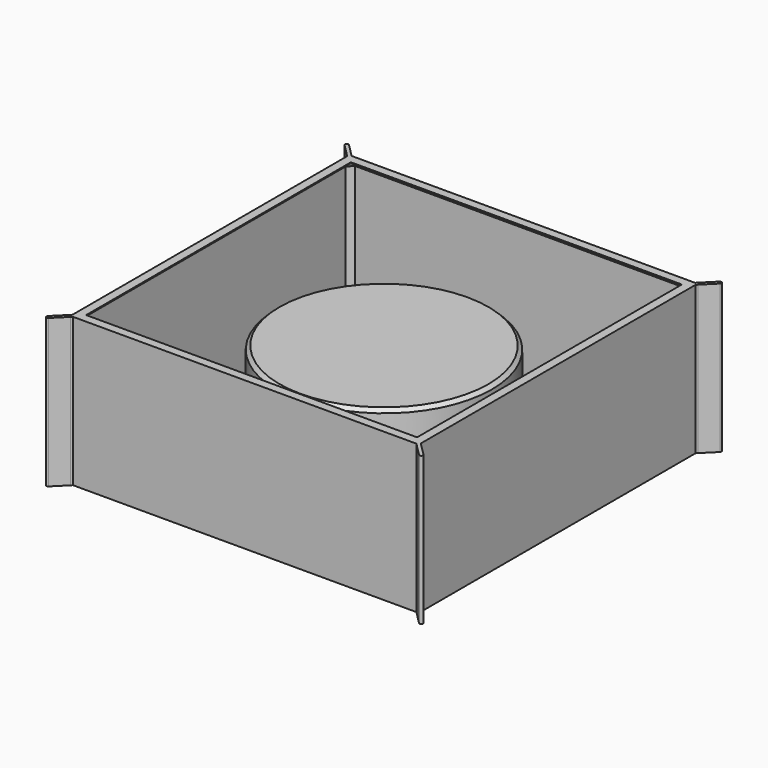
from build123d import *

# Parameters (mm, degrees)
F0_W             = 80
F0_H             = 80
F1_DEPTH         = 34
F2_T             = -0.8
F3_R             = 25
F4_DEPTH         = 24
F4_TAPER         = 0.5
F5_T1_DEPTH      = 78.4
F5_T3_DEPTH      = 78.4
F6_W             = 80
F6_H             = 80
F6_W_2           = 76
F6_H_2           = 76
F7_DEPTH         = 0.05
F8_SIZE          = 1.19999
F11_DEPTH        = 34.05
F11_COPIES_COUNT = 4


# Not quite as in the source:
# - a fillet or chamfer that OpenCascade refuses, or shapes differently, is made with other operations: its cross-section is extruded or revolved along the edge and cut away or added
# - a fillet or chamfer is up to 0.001 mm smaller than in the source, because OpenCascade refuses the exact size
# - a pattern or mirror of a feature is missing from the dataset's text; its kind, count and spacing are read off the source's solid


with BuildPart() as f1:
    # F0 (on Top) → F1 (new body)
    with BuildSketch(Plane.XY):
        Rectangle(F0_W, F0_H)
    extrude(amount=F1_DEPTH)

    # F2
    f2_openings = [f1.faces().sort_by_distance(p)[0] for p in [
        (0, 0, 34),
    ]]
    offset(amount=F2_T, openings=f2_openings)

    # F3 (on face) → F4 (join)
    with BuildSketch(Plane.XY.offset(0.8)):
        Circle(F3_R)
    extrude(amount=F4_DEPTH, taper=F4_TAPER)

    # F5: chamfer of 1.2 on 5 edges, made by hand

    # F5_s2 → F5_t1 (join)
    with BuildSketch(Plane.XZ.offset(-39.2)):
        Polygon((-39.2, 2), (-38, 0.8), (-39.2, 0.8), align=None)
        Polygon((39.2, 2), (38, 0.8), (39.2, 0.8), align=None)
    extrude(amount=F5_T1_DEPTH)

    # F5_s4 → F5_t3 (join)
    with BuildSketch(Plane.YZ.offset(-39.2)):
        Polygon((-39.2, 2), (-38, 0.8), (-39.2, 0.8), align=None)
        Polygon((39.2, 2), (38, 0.8), (39.2, 0.8), align=None)
    extrude(amount=F5_T3_DEPTH)

    # F5_s5 → F5_t6 (revolve)
    with BuildSketch(Plane.XZ):
        Polygon((26.1895734527, 0.8), (24.989619145, 1.9895281574), (25, 0.8), align=None)
    revolve(axis=Axis((0, 0, 0.8), (0, 0, -1)))

    # F6 (on face) → F7 (join)
    with BuildSketch(Plane.XY.offset(34)):
        Rectangle(F6_W, F6_H)
        Rectangle(F6_W_2, F6_H_2, mode=Mode.SUBTRACT)
    extrude(amount=F7_DEPTH)

    # F8 (size 1.2 in the source; OpenCascade refuses exactly that, so slightly less here)
    f8_edges = [f1.edges().sort_by_distance(p)[0] for p in [
        (0, -39.2, 34),
        (-39.2, 0, 34),
        (-39.2, -39.2, 18),
        (-39.2, 39.2, 18),
        (0, 39.2, 34),
        (39.2, 0, 34),
        (39.2, 39.2, 18),
        (39.2, -39.2, 18),
    ]]
    chamfer(f8_edges, length=F8_SIZE)

    # F9: chamfer of 0.8 on 1 edges, made by hand

    # F9_s1 → F9_t2 (revolve, cut)
    with BuildSketch(Plane.XZ):
        Polygon((24.7975364014, 24.0000304615), (23.990555173, 24.8), (24.790555173, 24.8), align=None)
    revolve(axis=Axis((0, 0, 24.8), (0, 0, -1)), mode=Mode.SUBTRACT)

    # F10 (on face) → F11 (join, through all)
    with BuildSketch(Plane(origin=(0, 0, 0), x_dir=(1, 0, 0), z_dir=(0, 0, -1))):
        with BuildLine():
            Line((-39.1612012219, 39.7268866468), (-39.7171572875, 40.2828427125))
            ThreePointArc((-39.7171572875, 40.2828427125), (-39.7171572875, 39.7171572875), (-40.2828427125, 39.7171572875))
            Line((-40.2828427125, 39.7171572875), (-39.7268866468, 39.1612012219))
            Line((-39.7268866468, 39.1612012219), (-39.1612012219, 39.7268866468))
        make_face()
        with BuildLine():
            ThreePointArc((-40.2828427125, 39.7171572875), (-39.7171572875, 39.7171572875), (-39.7171572875, 40.2828427125))
            Line((-39.7171572875, 40.2828427125), (-42.5455844123, 43.1112698372))
            ThreePointArc((-42.5455844123, 43.1112698372), (-43.1112698372, 43.1112698372), (-43.1112698372, 42.5455844123))
            Line((-43.1112698372, 42.5455844123), (-40.2828427125, 39.7171572875))
        make_face()
    f11 = extrude(amount=-F11_DEPTH)

    # F11_copies: F11 ×4 about axis
    f11_copies_axis = Axis((0, 0, 0), (0, 0, 1))
    for i in range(1, F11_COPIES_COUNT):
        add(f11.rotate(f11_copies_axis, i * 360 / F11_COPIES_COUNT))

    # F12 (on Front) → F13 (revolve, cut)
    with BuildSketch(Plane.XZ):
        Polygon((-23.9975059387, 24.0000304615), (-24.2264749318, -2.2372173829), (0, -2.2372173829), (0, 24.0000304615), align=None)
    revolve(axis=Axis((0, 0, 10.8814065393), (0, 0, 1)), mode=Mode.SUBTRACT)


solid = f1.part
